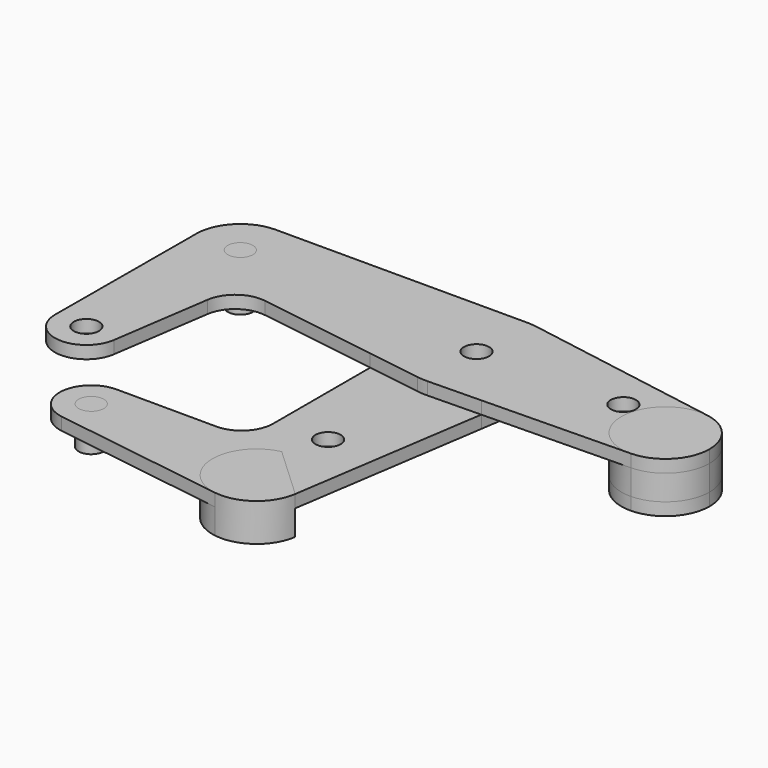
from build123d import *

# Parameters (mm, degrees)
F0_R     = 3.175
F1_DEPTH = 3.175
F2_DEPTH = 3.175
F4_R     = 3.175
F6_DEPTH = 9.525
F3_R     = 3.175


# Not quite as in the source:
# - a pattern or mirror of a feature is missing from the dataset's text; its kind, count and spacing are read off the source's solid


with BuildPart() as f1:
    # F0 (on Top) → F1 (new body)
    with BuildSketch(Plane.XY):
        with BuildLine():
            ThreePointArc((-15.875, 0), (-11.2253201513, 11.2253201513), (0, 15.875))
            Line((0, 15.875), (-63.3211543937, 15.875))
            ThreePointArc((-63.3211543937, 15.875), (-55.4634302878, 12.6202241059), (-52.2086543937, 4.7625))
            ThreePointArc((-52.2086543937, 4.7625), (-63.3410515432, -6.3499821869), (-74.4335831412, 4.8022942352))
            Line((-74.4335831412, 4.8022942352), (-74.5923534991, -39.5338836219))
            ThreePointArc((-74.5923534991, -39.5338836219), (-66.6406921441, -31.6248207993), (-58.7174043937, -39.5623080756))
            ThreePointArc((-58.7174043937, -39.5623080756), (-58.7387068636, -40.1434474), (-58.8024999312, -40.7214674292))
            Line((-58.8024999312, -40.7214674292), (-55.1216121776, -15.7863113327))
            ThreePointArc((-55.1216121776, -15.7863113327), (-51.9856201231, -10.5565144679), (-46.0674725884, -9.0865650912))
            Line((-46.0674725884, -9.0865650912), (-15.875, -13.6540649408))
            Line((-15.875, -13.6540649408), (-15.875, 0))
        make_face()
        with BuildLine():
            ThreePointArc((-52.2086543937, 4.7625), (-55.4634302878, 12.6202241059), (-63.3211543937, 15.875))
            ThreePointArc((-63.3211543937, 15.875), (-71.1647964945, 12.6342809195), (-74.4335831412, 4.8022942352))
            ThreePointArc((-74.4335831412, 4.8022942352), (-63.3410515432, -6.3499821869), (-52.2086543937, 4.7625))
        make_face()
        with Locations((-63.3211543937, 4.7625)):
            Circle(F0_R, mode=Mode.SUBTRACT)
        with BuildLine():
            ThreePointArc((15.69640625, -2.3745432898), (15.8302885984, -1.190625), (15.875, 0))
            ThreePointArc((15.875, 0), (12.1324662265, 10.238109604), (2.6694707699, 15.6489472748))
            ThreePointArc((2.6694707699, 15.6489472748), (1.3395124137, 15.8183858688), (0, 15.875))
            ThreePointArc((0, 15.875), (-11.2253201513, 11.2253201513), (-15.875, 0))
            ThreePointArc((-15.875, 0), (-12.0356034274, -10.3518054047), (-2.3745432898, -15.69640625))
            ThreePointArc((-2.3745432898, -15.69640625), (-1.0416321888, -15.8407899861), (0.2987083423, -15.8721894623))
            ThreePointArc((0.2987083423, -15.8721894623), (10.4645848343, -11.9376752027), (15.69640625, -2.3745432898))
        make_face()
        Circle(F0_R, mode=Mode.SUBTRACT)
        with BuildLine():
            ThreePointArc((61.769423515, -3.81), (59.1496498735, 3.3566767228), (52.5255530539, 7.1442630923))
            ThreePointArc((52.5255530539, 7.1442630923), (39.5757214961, -2.9765625), (50.8660193546, -14.9205326236))
            ThreePointArc((50.8660193546, -14.9205326236), (58.5882296422, -11.5934464966), (61.769423515, -3.81))
        make_face()
        with Locations((50.656923515, -3.81)):
            Circle(F0_R, mode=Mode.SUBTRACT)
        with BuildLine():
            ThreePointArc((2.6694707699, 15.6489472748), (12.1324662265, 10.238109604), (15.875, 0))
            ThreePointArc((15.875, 0), (15.8302885984, -1.190625), (15.69640625, -2.3745432898))
            Line((15.69640625, -2.3745432898), (13.6926228472, -15.6201212767))
            Line((13.6926228472, -15.6201212767), (50.8660193546, -14.9205326236))
            ThreePointArc((50.8660193546, -14.9205326236), (39.5757214961, -2.9765625), (52.5255530539, 7.1442630923))
            Line((52.5255530539, 7.1442630923), (2.6694707699, 15.6489472748))
        make_face()
        with BuildLine():
            ThreePointArc((36.4223280073, -2.73939), (34.501219564, 2.7543996496), (39.8354530073, 0.4266677197))
            ThreePointArc((39.8354530073, 0.4266677197), (38.8196864505, -1.9010642102), (36.4223280073, -2.73939))
        make_face(mode=Mode.SUBTRACT)
        with BuildLine():
            Line((13.6926228472, -15.6201212767), (15.69640625, -2.3745432898))
            ThreePointArc((15.69640625, -2.3745432898), (10.4645848343, -11.9376752027), (0.2987083423, -15.8721894623))
            Line((0.2987083423, -15.8721894623), (13.6926228472, -15.6201212767))
        make_face()
        with BuildLine():
            ThreePointArc((-2.3745432898, -15.69640625), (-12.0356034274, -10.3518054047), (-15.875, 0))
            Line((-15.875, 0), (-15.875, -13.6540649408))
            Line((-15.875, -13.6540649408), (-2.3745432898, -15.69640625))
        make_face()
        with BuildLine():
            ThreePointArc((-58.7174043937, -39.5623080756), (-66.6406921441, -31.6248207993), (-74.5923534991, -39.5338836219))
            ThreePointArc((-74.5923534991, -39.5338836219), (-67.2502168937, -47.4774523748), (-58.8024999312, -40.7214674292))
            ThreePointArc((-58.8024999312, -40.7214674292), (-58.7387068636, -40.1434474), (-58.7174043937, -39.5623080756))
        make_face()
        with Locations((-66.6549043937, -39.5623080756)):
            Circle(F0_R, mode=Mode.SUBTRACT)
    extrude(amount=F1_DEPTH)


with BuildPart() as f2:
    # F0 (on Top) → F2 (new body)
    with BuildSketch(Plane.XY):
        with BuildLine():
            Line((13.6926228472, -15.6201212767), (0.2987083423, -15.8721894623))
            ThreePointArc((0.2987083423, -15.8721894623), (-1.0416321888, -15.8407899861), (-2.3745432898, -15.69640625))
            Line((-2.3745432898, -15.69640625), (-15.875, -13.6540649408))
            Line((-15.875, -13.6540649408), (-15.875, -44.1900675587))
            ThreePointArc((-15.875, -44.1900675587), (-18.213634337, -49.8217645365), (-23.8536699328, -52.1402165826))
            Line((-23.8536699328, -52.1402165826), (-49.0588836219, -52.0499552883))
            ThreePointArc((-49.0588836219, -52.0499552883), (-43.4646074188, -54.3848028931), (-41.1498080756, -59.9874043937))
            ThreePointArc((-41.1498080756, -59.9874043937), (-43.9006386779, -65.9959289055), (-50.2464674292, -67.8398088562))
            Line((-50.2464674292, -67.8398088562), (-6.385323095, -74.3145206412))
            ThreePointArc((-6.385323095, -74.3145206412), (-12.0238371567, -54.9092200771), (6.35, -63.3211543937))
            ThreePointArc((6.35, -63.3211543937), (6.3187020189, -64.1545918937), (6.224984375, -64.9833346965))
            Line((6.224984375, -64.9833346965), (13.6926228472, -15.6201212767))
        make_face()
        with Locations((-3.213735, -42.7291149849)):
            Circle(F0_R, mode=Mode.SUBTRACT)
        with BuildLine():
            ThreePointArc((-49.0588836219, -52.0499552883), (-57.0024523748, -59.3920918937), (-50.2464674292, -67.8398088562))
            ThreePointArc((-50.2464674292, -67.8398088562), (-43.9006386779, -65.9959289055), (-41.1498080756, -59.9874043937))
            ThreePointArc((-41.1498080756, -59.9874043937), (-43.4646074188, -54.3848028931), (-49.0588836219, -52.0499552883))
        make_face()
        with Locations((-49.0873080756, -59.9874043937)):
            Circle(F0_R, mode=Mode.SUBTRACT)
        with BuildLine():
            ThreePointArc((-6.385323095, -74.3145206412), (1.847490772, -72.253997068), (6.224984375, -64.9833346965))
            ThreePointArc((6.224984375, -64.9833346965), (6.3187020189, -64.1545918937), (6.35, -63.3211543937))
            ThreePointArc((6.35, -63.3211543937), (-12.0238371567, -54.9092200771), (-6.385323095, -74.3145206412))
        make_face()
        with Locations((-4.7625, -63.3211543937)):
            Circle(F0_R, mode=Mode.SUBTRACT)
        with BuildLine():
            ThreePointArc((15.69640625, -2.3745432898), (15.8302885984, -1.190625), (15.875, 0))
            ThreePointArc((15.875, 0), (12.1324662265, 10.238109604), (2.6694707699, 15.6489472748))
            ThreePointArc((2.6694707699, 15.6489472748), (1.3395124137, 15.8183858688), (0, 15.875))
            ThreePointArc((0, 15.875), (-11.2253201513, 11.2253201513), (-15.875, 0))
            ThreePointArc((-15.875, 0), (-12.0356034274, -10.3518054047), (-2.3745432898, -15.69640625))
            ThreePointArc((-2.3745432898, -15.69640625), (-1.0416321888, -15.8407899861), (0.2987083423, -15.8721894623))
            ThreePointArc((0.2987083423, -15.8721894623), (10.4645848343, -11.9376752027), (15.69640625, -2.3745432898))
        make_face()
        Circle(F0_R, mode=Mode.SUBTRACT)
        with BuildLine():
            Line((13.6926228472, -15.6201212767), (15.69640625, -2.3745432898))
            ThreePointArc((15.69640625, -2.3745432898), (10.4645848343, -11.9376752027), (0.2987083423, -15.8721894623))
            Line((0.2987083423, -15.8721894623), (13.6926228472, -15.6201212767))
        make_face()
        with BuildLine():
            ThreePointArc((-2.3745432898, -15.69640625), (-12.0356034274, -10.3518054047), (-15.875, 0))
            Line((-15.875, 0), (-15.875, -13.6540649408))
            Line((-15.875, -13.6540649408), (-2.3745432898, -15.69640625))
        make_face()
    extrude(amount=-F2_DEPTH)


with BuildPart() as f6:
    # F4 (on face) → F6 (new body, through all)
    with BuildSketch(Plane.XY):
        with Locations((-49.0873080756, -59.9874043937)):
            Circle(F4_R)
    extrude(amount=-F6_DEPTH)


with BuildPart() as f6b:
    # F4 (on face) → F6, piece 2 (new body, through all)
    with BuildSketch(Plane.XY):
        with BuildLine():
            ThreePointArc((-7.1087737889, -52.4591722745), (-15.8689168649, -63.6887964396), (-6.385323095, -74.3145206412))
            ThreePointArc((-6.385323095, -74.3145206412), (1.847490772, -72.253997068), (6.224984375, -64.9833346965))
            ThreePointArc((6.224984375, -64.9833346965), (6.232010065, -64.9362100216), (6.2388336409, -64.8890556569))
            Line((6.2388336409, -64.8890556569), (-7.1087737889, -52.4591722745))
        make_face()
        with Locations((-4.7625, -63.3211543937)):
            Circle(F4_R, mode=Mode.SUBTRACT)
        with Locations((-4.7625, -63.3211543937)):
            Circle(F4_R)
    extrude(amount=-F6_DEPTH)


with BuildPart() as f6c:
    # F3 (on face) → F6, piece 3 (new body, through all)
    with BuildSketch(Plane.XY.offset(3.175)):
        with Locations((-63.3211543937, 4.7625)):
            Circle(F3_R)
    extrude(amount=-F6_DEPTH)

    # F6_3_copies: F6c across plane


with BuildPart() as f6d:
    # F3 (on face) → F6, piece 4 (new body, through all)
    with BuildSketch(Plane.XY.offset(3.175)):
        with BuildLine():
            ThreePointArc((50.8660193546, -14.9205326236), (58.5882296422, -11.5934464966), (61.769423515, -3.81))
            ThreePointArc((61.769423515, -3.81), (59.1496498735, 3.3566767228), (52.5255530539, 7.1442630923))
            ThreePointArc((52.5255530539, 7.1442630923), (39.5757214961, -2.9765625), (50.8660193546, -14.9205326236))
        make_face()
        with Locations((50.656923515, -3.81)):
            Circle(F3_R, mode=Mode.SUBTRACT)
        with Locations((50.656923515, -3.81)):
            Circle(F3_R)
    extrude(amount=-F6_DEPTH)

    # F6_4_copies: F6d across plane


with BuildPart() as f6c_1:
    add(f6c.part)
    add(f6c.part.mirror(Plane(origin=(0, 0, -3.175), x_dir=(-1, 0, 0), z_dir=(0, 0, -1))))


with BuildPart() as f6d_1:
    add(f6d.part)
    add(f6d.part.mirror(Plane(origin=(0, 0, -3.175), x_dir=(-1, 0, 0), z_dir=(0, 0, -1))))


solid = Compound([f1.part, f2.part, f6.part, f6b.part, f6c_1.part, f6d_1.part])
